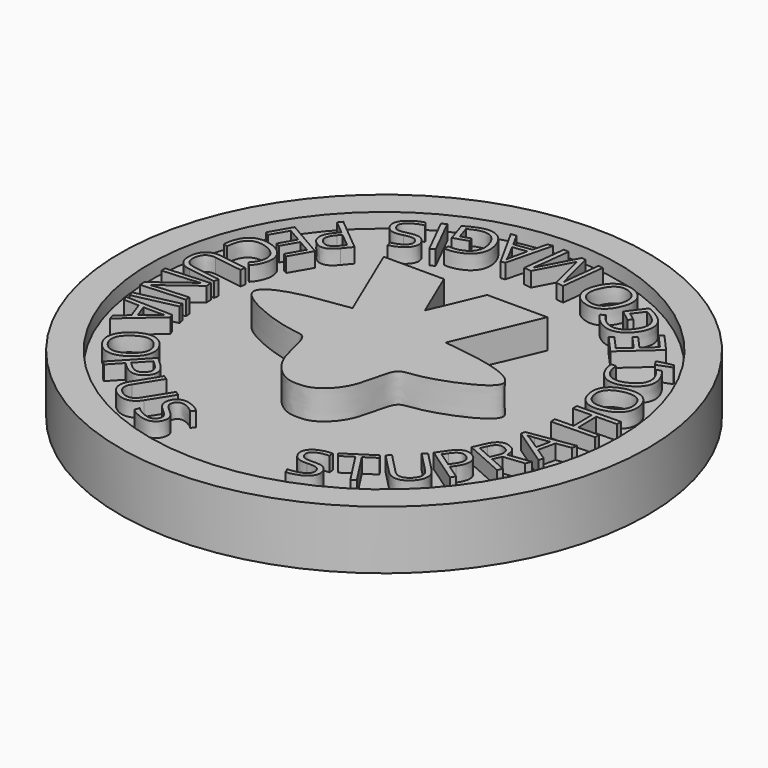
from build123d import *

# Parameters (mm, degrees)
F2_R          = 9
F3_DEPTH      = 2
F4_R          = 8
F5_DEPTH      = 0.5
F6_R          = 8
F7_DEPTH      = 0.5
F8_TEXT_SIZE  = 11.8055555556
F9_DEPTH      = 0.5
F11_DEPTH     = 1
F12_TEXT_SIZE = 2.0833333333
F13_DEPTH     = 0.5


# Not quite as in the source:
# - Text() gives the source's letters only with a copy of the font that has no kerning and outlines rounded to 1/6400 em; it was checked with that copy


with BuildPart() as f3:
    # F2 (on Top) → F3 (new body)
    with BuildSketch(Plane.XY):
        Circle(F2_R)
    extrude(amount=F3_DEPTH)

    # F4 (on face) → F5 (cut)
    with BuildSketch(Plane.XY.offset(2)):
        Circle(F4_R)
    extrude(amount=-F5_DEPTH, mode=Mode.SUBTRACT)

    # F6 (on face) → F7 (cut)
    with BuildSketch(Plane(origin=(0, 0, 0), x_dir=(1, 0, 0), z_dir=(0, 0, -1))):
        Circle(F6_R)
    extrude(amount=-F7_DEPTH, mode=Mode.SUBTRACT)

    # F8 (on face) → F9 (join)
    with BuildSketch(Plane(origin=(0, 0, 0.5), x_dir=(1, 0, 0), z_dir=(0, 0, -1))):
        with Locations((-3.6431966146, -4.25)):
            Text('1', F8_TEXT_SIZE, font='Open Sans', text_align=(TextAlign.LEFT, TextAlign.BOTTOM))
    extrude(amount=F9_DEPTH)

    # F10 (on face) → F11 (join)
    with BuildSketch(Plane.XY.offset(1.5)):
        with BuildLine():
            Line((0.7361412053, 3.471448), (0, 1.737208))
            Line((0, 1.737208), (-0.7361412053, 3.471448))
            Line((-0.7361412053, 3.471448), (-2.7898692053, 3.471448))
            Line((-2.7898692053, 3.471448), (-1.5882930619, 0.640712))
            add(Edge.make_bspline(
                [(-1.5882930619, 0.640712), (-2.288944, 0.53364), (-3.5094865455, 0.4309933697), (-4.8411924257, -0.4110598015), (-2.2223525913, -1.444643169), (-1.4478338187, -1.2881000832), (-1.3536249759, -2.8972097583), (-0.502673709, -3.6650017818), (-0.143104, -3.68), (0, -3.68)],
                knots=[0, 0, 0, 0, 0.1906946011, 0.3116321419, 0.5087037577, 0.6185878054, 0.772744227, 0.9107655949, 1, 1, 1, 1], degree=3))
            add(Edge.make_bspline(
                [(1.5882930619, 0.640712), (2.288944, 0.53364), (3.5094865455, 0.4309933697), (4.8411924257, -0.4110598015), (2.2223525913, -1.444643169), (1.4478338187, -1.2881000832), (1.3536249759, -2.8972097583), (0.502673709, -3.6650017818), (0.143104, -3.68), (0, -3.68)],
                knots=[0, 0, 0, 0, 0.1906946011, 0.3116321419, 0.5087037577, 0.6185878054, 0.772744227, 0.9107655949, 1, 1, 1, 1], degree=3))
            Line((1.5882930619, 0.640712), (2.7898692053, 3.471448))
            Line((2.7898692053, 3.471448), (0.7361412053, 3.471448))
        make_face()
    extrude(amount=F11_DEPTH)

    # F12 (on face) → F13 (join)
    with BuildSketch(Plane.XY.offset(1.5)):
        with Locations(Location((-3.6860037573, 6.5582555737), (0, 0, -146.1691486022))):
            Text('S', F12_TEXT_SIZE, font='Open Sans', text_align=(TextAlign.LEFT, TextAlign.BOTTOM))
        with Locations(Location((-2.915357097, 5.2503641491), (0, 0, 26.5970945547))):
            Text('I', F12_TEXT_SIZE, font='Open Sans', text_align=(TextAlign.LEFT, TextAlign.BOTTOM))
        with Locations(Location((-1.5989614672, 7.3658220214), (0, 0, -162.0442109826))):
            Text('G', F12_TEXT_SIZE, font='Open Sans', text_align=(TextAlign.LEFT, TextAlign.BOTTOM))
        with Locations(Location((-0.2584384166, 7.5306931413), (0, 0, -172.5))):
            Text('A', F12_TEXT_SIZE, font='Open Sans', text_align=(TextAlign.LEFT, TextAlign.BOTTOM))
        with Locations(Location((1.7672024578, 7.3449495938), (0, 0, 173.3615474995))):
            Text('M', F12_TEXT_SIZE, font='Open Sans', text_align=(TextAlign.LEFT, TextAlign.BOTTOM))
        with Locations(Location((-5.3610910866, 5.2839319945), (0, 0, -129.6976045126))):
            Text('P', F12_TEXT_SIZE, font='Open Sans', text_align=(TextAlign.LEFT, TextAlign.BOTTOM))
        with Locations(Location((-6.2048682948, 4.2533548522), (0, 0, -119.9753197604))):
            Text('E', F12_TEXT_SIZE, font='Open Sans', text_align=(TextAlign.LEFT, TextAlign.BOTTOM))
        with Locations(Location((-6.7848294721, 3.2706708439), (0, 0, -110.4523635335))):
            Text('C', F12_TEXT_SIZE, font='Open Sans', text_align=(TextAlign.LEFT, TextAlign.BOTTOM))
        with Locations(Location((-7.3110490051, 1.8257427573), (0, 0, -98.4523635335))):
            Text('U', F12_TEXT_SIZE, font='Open Sans', text_align=(TextAlign.LEFT, TextAlign.BOTTOM))
        with Locations(Location((-7.5326887018, 0.2684732903), (0, 0, -86.3257029841))):
            Text('N', F12_TEXT_SIZE, font='Open Sans', text_align=(TextAlign.LEFT, TextAlign.BOTTOM))
        with Locations(Location((-7.3792511523, -1.3646549501), (0, 0, -77.5662367398))):
            Text('I', F12_TEXT_SIZE, font='Open Sans', text_align=(TextAlign.LEFT, TextAlign.BOTTOM))
        with Locations(Location((-7.2999590891, -1.8678134013), (0, 0, -70.1133597403))):
            Text('A', F12_TEXT_SIZE, font='Open Sans', text_align=(TextAlign.LEFT, TextAlign.BOTTOM))
        with Locations(Location((-6.574935783, -3.6993079909), (0, 0, -54.4324233574))):
            Text('O', F12_TEXT_SIZE, font='Open Sans', text_align=(TextAlign.LEFT, TextAlign.BOTTOM))
        with Locations(Location((-5.6031886019, -5.0264811204), (0, 0, -43.2184079253))):
            Text('P', F12_TEXT_SIZE, font='Open Sans', text_align=(TextAlign.LEFT, TextAlign.BOTTOM))
        with Locations(Location((-4.6067339389, -5.9634534111), (0, 0, -32.1168993039))):
            Text('U', F12_TEXT_SIZE, font='Open Sans', text_align=(TextAlign.LEFT, TextAlign.BOTTOM))
        with Locations(Location((-3.1868503577, -6.8147872062), (0, 0, -20.5694446729))):
            Text('S', F12_TEXT_SIZE, font='Open Sans', text_align=(TextAlign.LEFT, TextAlign.BOTTOM))
        with Locations(Location((2.2357243324, -7.1832358014), (0, 0, 21.7814442764))):
            Text('S', F12_TEXT_SIZE, font='Open Sans', text_align=(TextAlign.LEFT, TextAlign.BOTTOM))
        with Locations(Location((3.5395308549, -6.6425765056), (0, 0, 32.8839352993))):
            Text('T', F12_TEXT_SIZE, font='Open Sans', text_align=(TextAlign.LEFT, TextAlign.BOTTOM))
        with Locations(Location((4.7029427583, -5.8878776807), (0, 0, 44.1850972077))):
            Text('U', F12_TEXT_SIZE, font='Open Sans', text_align=(TextAlign.LEFT, TextAlign.BOTTOM))
        with Locations(Location((5.8164810771, -4.7780522016), (0, 0, 55.4850972077))):
            Text('P', F12_TEXT_SIZE, font='Open Sans', text_align=(TextAlign.LEFT, TextAlign.BOTTOM))
        with Locations(Location((6.56839761, -3.6861024906), (0, 0, 65.9837331588))):
            Text('R', F12_TEXT_SIZE, font='Open Sans', text_align=(TextAlign.LEFT, TextAlign.BOTTOM))
        with Locations(Location((7.1557863146, -2.3606888451), (0, 0, 77.2768077788))):
            Text('A', F12_TEXT_SIZE, font='Open Sans', text_align=(TextAlign.LEFT, TextAlign.BOTTOM))
        with Locations(Location((7.5124764219, -0.593299799), (0, 0, 91.0768077788))):
            Text('H', F12_TEXT_SIZE, font='Open Sans', text_align=(TextAlign.LEFT, TextAlign.BOTTOM))
        with Locations(Location((7.4753607344, 1.0166818835), (0, 0, 103.9487794663))):
            Text('O', F12_TEXT_SIZE, font='Open Sans', text_align=(TextAlign.LEFT, TextAlign.BOTTOM))
        with Locations(Location((7.0452060298, 2.6638826425), (0, 0, 115.9965752941))):
            Text('C', F12_TEXT_SIZE, font='Open Sans', text_align=(TextAlign.LEFT, TextAlign.BOTTOM))
        with Locations(Location((6.437618423, 3.8563204275), (0, 0, 122.8568259107))):
            Text(',', F12_TEXT_SIZE, font='Open Sans', text_align=(TextAlign.LEFT, TextAlign.BOTTOM))
        with Locations(Location((5.9760025941, 4.5693337644), (0, 0, 131.8568259107))):
            Text('E', F12_TEXT_SIZE, font='Open Sans', text_align=(TextAlign.LEFT, TextAlign.BOTTOM))
        with Locations(Location((5.1135922216, 5.5374350034), (0, 0, 142.9869342885))):
            Text('G', F12_TEXT_SIZE, font='Open Sans', text_align=(TextAlign.LEFT, TextAlign.BOTTOM))
        with Locations(Location((3.7540905164, 6.5438111645), (0, 0, 156.3615474995))):
            Text('O', F12_TEXT_SIZE, font='Open Sans', text_align=(TextAlign.LEFT, TextAlign.BOTTOM))
    extrude(amount=F13_DEPTH)


solid = f3.part
